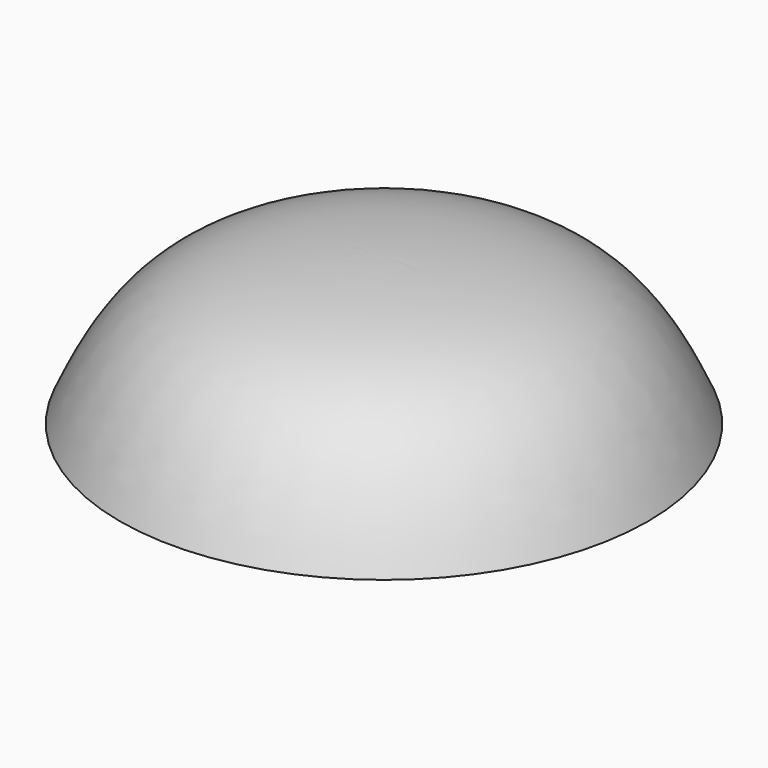
from build123d import *


# Not quite as in the source:
# - the program builds the solid bodies; features that only make, move or delete a surface that nothing else refers to are left out


with BuildPart() as f3:
    # F2 (on Front) → F3 (revolve)
    with BuildSketch(Plane.XZ):
        with BuildLine():
            add(Edge.make_bspline(
                [(0, 5.132293878), (2.2821105085, 5.1114950329), (2.9520839453, 4.6002417803), (3.6044276785, 3.100293878)],
                knots=[0, 0, 0, 0, 4.1377436955, 4.1377436955, 4.1377436955, 4.1377436955], degree=3))
            Line((0, 5.132293878), (0, 3.100293878))
            Line((0, 3.100293878), (3.6044276785, 3.100293878))
        make_face()
    revolve(axis=Axis((0, 0, 4.116293878), (0, 0, -1)))


solid = f3.part
